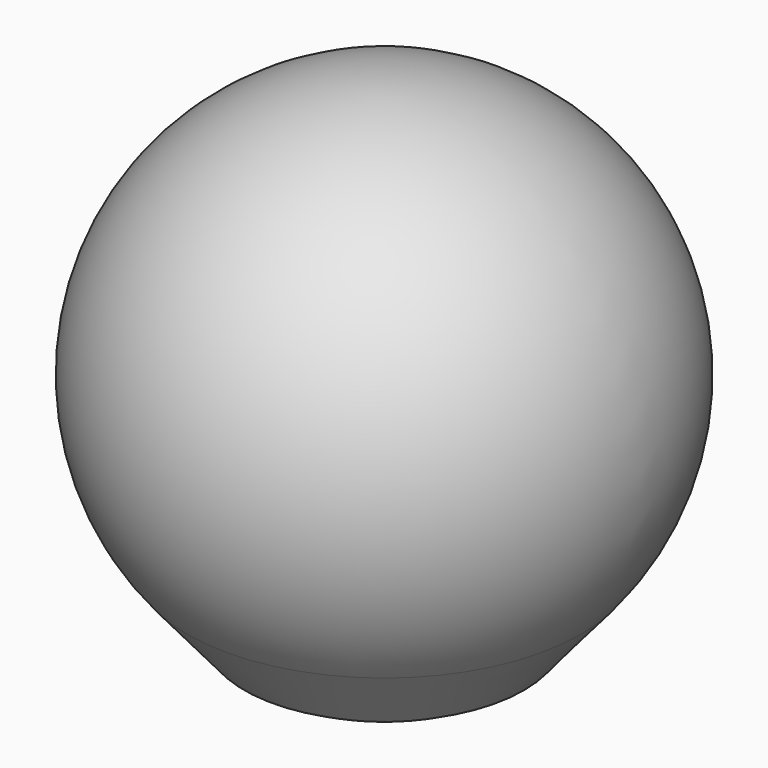
from build123d import *

# Parameters (mm, degrees)
F2_R     = 1.143
F3_DEPTH = 12.7
F4_SIZE  = 1.016
F7_R     = 2.286
F8_DEPTH = 25.4


# Not quite as in the source:
# - a feature names something its author has since deleted; it is built from what else it names


with BuildPart() as f1:
    # F0 (on Front) → F1 (revolve)
    with BuildSketch(Plane.XZ):
        with BuildLine():
            Line((22.1477128222, 0), (31.1320461684, 10.7071115423))
            ThreePointArc((31.1320461684, 10.7071115423), (36.8323484652, 54.0052061571), (0, 77.47))
            Line((0, 77.47), (0, 0))
            Line((0, 0), (22.1477128222, 0))
        make_face()
    revolve(axis=Axis((0, 0, -28.7515761617), (0, 0, -1)))

    # F2 (on face) → F3 (cut)
    with BuildSketch(Plane(origin=(0, 0, 0), x_dir=(1, 0, 0), z_dir=(0, 0, -1))):
        Circle(F2_R)
    extrude(amount=-F3_DEPTH, mode=Mode.SUBTRACT)

    # F4
    f4_edges = [f1.edges().sort_by_distance(p)[0] for p in [
        (-1.143, 0, 12.7),
    ]]
    chamfer(f4_edges, length=F4_SIZE)


with BuildPart() as f6:
    # F5 (on Front) → F6 (revolve)
    with BuildSketch(Plane.XZ):
        with BuildLine():
            Line((0, -1.016), (0, -6.1463898351))
            ThreePointArc((0, -6.1463898351), (11.4923810768, -4.5812938755), (22.1477128222, 0))
            Line((22.1477128222, 0), (15.7977128222, 0))
            Line((15.7977128222, 0), (15.7977128222, -1.016))
            Line((15.7977128222, -1.016), (0, -1.016))
        make_face()
    revolve(axis=Axis((0, 0, -28.7515761617), (0, 0, -1)))

    # F7 (on face) → F8 (cut)
    with BuildSketch(Plane.XY.offset(-1.016)):
        Circle(F7_R)
    extrude(amount=-F8_DEPTH, mode=Mode.SUBTRACT)


solid = Compound([f1.part, f6.part])
